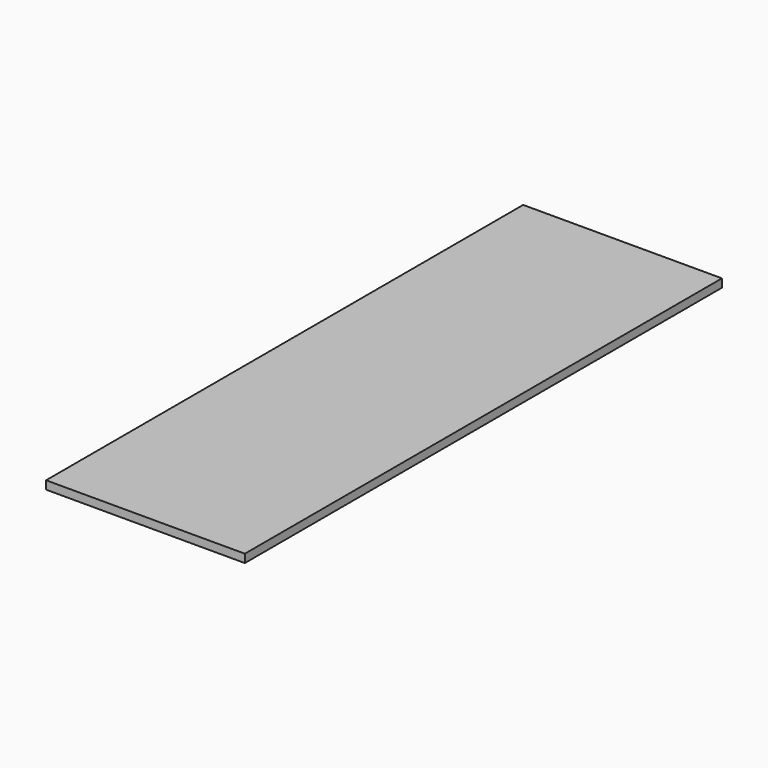
from build123d import *

# Parameters (mm, degrees)
F0_W     = 304.8
F0_H     = 914.4
F1_DEPTH = 12.7


# Not quite as in the source:
# - a feature names something its author has since deleted; it is built from what else it names


with BuildPart() as f1:
    # F0 (on Top) → F1 (new body)
    with BuildSketch(Plane.XY):
        Rectangle(F0_W, F0_H)
    extrude(amount=F1_DEPTH)


solid = f1.part
